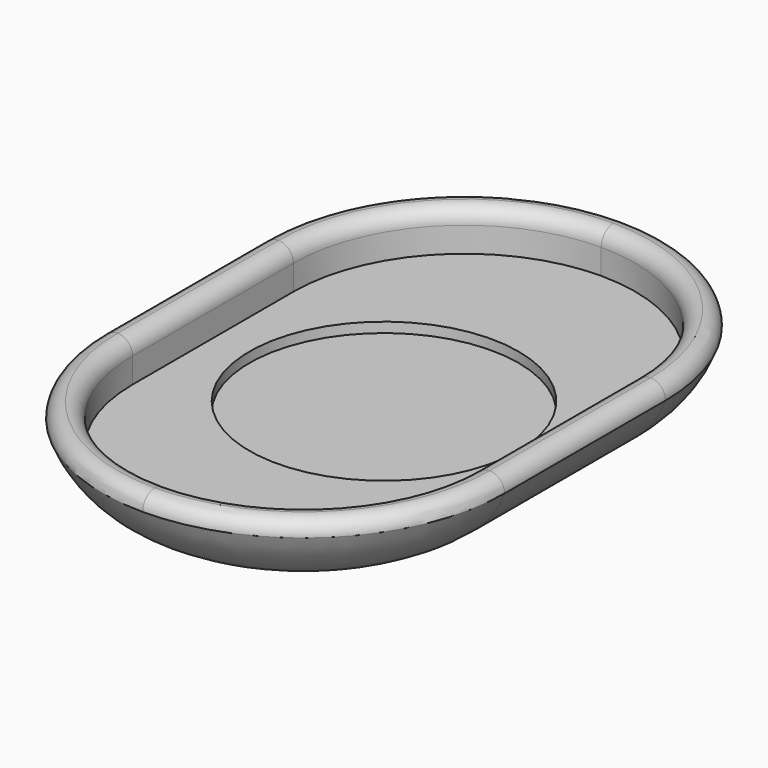
from build123d import *

# Parameters (mm, degrees)
F0_R        = 13.3863330109
F1_DEPTH    = 4
F2_DEPTH    = 8
F3_DEPTH    = 3
F4_R        = 1.49999
F5_T1_DEPTH = 20
F5_T4_ANGLE = 180
F5_T6_ANGLE = 180


# Not quite as in the source:
# - a fillet or chamfer that OpenCascade refuses, or shapes differently, is made with other operations: its cross-section is extruded or revolved along the edge and cut away or added
# - a fillet or chamfer is up to 0.001 mm smaller than in the source, because OpenCascade refuses the exact size


with BuildPart() as f1:
    # F0 (on Top) → F1 (new body)
    with BuildSketch(Plane.XY):
        with BuildLine():
            ThreePointArc((0, -30), (14.1421356237, -24.1421356237), (20, -10))
            Line((20, -10), (20, 10))
            ThreePointArc((20, 10), (14.1421356237, 24.1421356237), (0, 30))
            ThreePointArc((0, 30), (-14.1421356237, 24.1421356237), (-20, 10))
            Line((-20, 10), (-20, -10))
            ThreePointArc((-20, -10), (-14.1421356237, -24.1421356237), (0, -30))
        make_face()
        with BuildLine():
            Line((17, 10), (17, -10))
            ThreePointArc((17, -10), (12.0208152802, -22.0208152802), (0, -27))
            ThreePointArc((0, -27), (-12.0208152802, -22.0208152802), (-17, -10))
            Line((-17, -10), (-17, 10))
            ThreePointArc((-17, 10), (-12.0208152802, 22.0208152802), (0, 27))
            ThreePointArc((0, 27), (12.0208152802, 22.0208152802), (17, 10))
        make_face(mode=Mode.SUBTRACT)
        with BuildLine():
            ThreePointArc((0, -27), (12.0208152802, -22.0208152802), (17, -10))
            Line((17, -10), (17, 10))
            ThreePointArc((17, 10), (12.0208152802, 22.0208152802), (0, 27))
            ThreePointArc((0, 27), (-12.0208152802, 22.0208152802), (-17, 10))
            Line((-17, 10), (-17, -10))
            ThreePointArc((-17, -10), (-12.0208152802, -22.0208152802), (0, -27))
        make_face()
        Circle(F0_R, mode=Mode.SUBTRACT)
    extrude(amount=F1_DEPTH)

    # F0 (on Top) → F2 (join)
    with BuildSketch(Plane.XY):
        with BuildLine():
            ThreePointArc((0, -30), (14.1421356237, -24.1421356237), (20, -10))
            Line((20, -10), (20, 10))
            ThreePointArc((20, 10), (14.1421356237, 24.1421356237), (0, 30))
            ThreePointArc((0, 30), (-14.1421356237, 24.1421356237), (-20, 10))
            Line((-20, 10), (-20, -10))
            ThreePointArc((-20, -10), (-14.1421356237, -24.1421356237), (0, -30))
        make_face()
        with BuildLine():
            Line((17, 10), (17, -10))
            ThreePointArc((17, -10), (12.0208152802, -22.0208152802), (0, -27))
            ThreePointArc((0, -27), (-12.0208152802, -22.0208152802), (-17, -10))
            Line((-17, -10), (-17, 10))
            ThreePointArc((-17, 10), (-12.0208152802, 22.0208152802), (0, 27))
            ThreePointArc((0, 27), (12.0208152802, 22.0208152802), (17, 10))
        make_face(mode=Mode.SUBTRACT)
    extrude(amount=F2_DEPTH)

    # F0 (on Top) → F3 (join)
    with BuildSketch(Plane.XY):
        Circle(F0_R)
    extrude(amount=F3_DEPTH)

    # F4 (radius 1.5 in the source; OpenCascade refuses exactly that, so slightly less here)
    f4_edges = [f1.edges().sort_by_distance(p)[0] for p in [
        (17, 0, 8),
        (0, -27, 8),
        (0, 27, 8),
        (20, 0, 8),
        (0, -30, 8),
        (0, 30, 8),
        (-20, 0, 8),
        (-17, 0, 8),
    ]]
    fillet(f4_edges, radius=F4_R)

    # F5: fillet of radius 10 on 2 edges, made by hand

    # F5_s2 → F5_t1 (cut)
    with BuildSketch(Plane.XZ.offset(-10)):
        with BuildLine():
            ThreePointArc((-10.6324992661, 0), (-16.3333807769, 1.7841646803), (-20, 6.50001))
            Line((-20, 6.50001), (-20, 0))
            Line((-20, 0), (-10.6324992661, 0))
        make_face()
        with BuildLine():
            ThreePointArc((20, 6.50001), (16.3333807769, 1.7841646803), (10.6324992661, 0))
            Line((10.6324992661, 0), (20, 0))
            Line((20, 0), (20, 6.50001))
        make_face()
    extrude(amount=F5_T1_DEPTH, mode=Mode.SUBTRACT)

    # F5_s3 → F5_t4 (revolve, cut)
    with BuildSketch(Plane.XZ.offset(10)):
        with BuildLine():
            ThreePointArc((-20, 6.50001), (-16.3333807769, 1.7841646803), (-10.6324992661, 0))
            Line((-10.6324992661, 0), (-20, 0))
            Line((-20, 0), (-20, 6.50001))
        make_face()
    revolve(axis=Axis((0, -10, 0), (0, 0, 1)), revolution_arc=F5_T4_ANGLE, mode=Mode.SUBTRACT)

    # F5_s5 → F5_t6 (revolve, cut)
    with BuildSketch(Plane.XZ.offset(-10)):
        with BuildLine():
            ThreePointArc((10.6324992661, 0), (16.3333807769, 1.7841646803), (20, 6.50001))
            Line((20, 6.50001), (20, 0))
            Line((20, 0), (10.6324992661, 0))
        make_face()
    revolve(axis=Axis((0, 10, 0), (0, 0, 1)), revolution_arc=F5_T6_ANGLE, mode=Mode.SUBTRACT)


solid = f1.part
